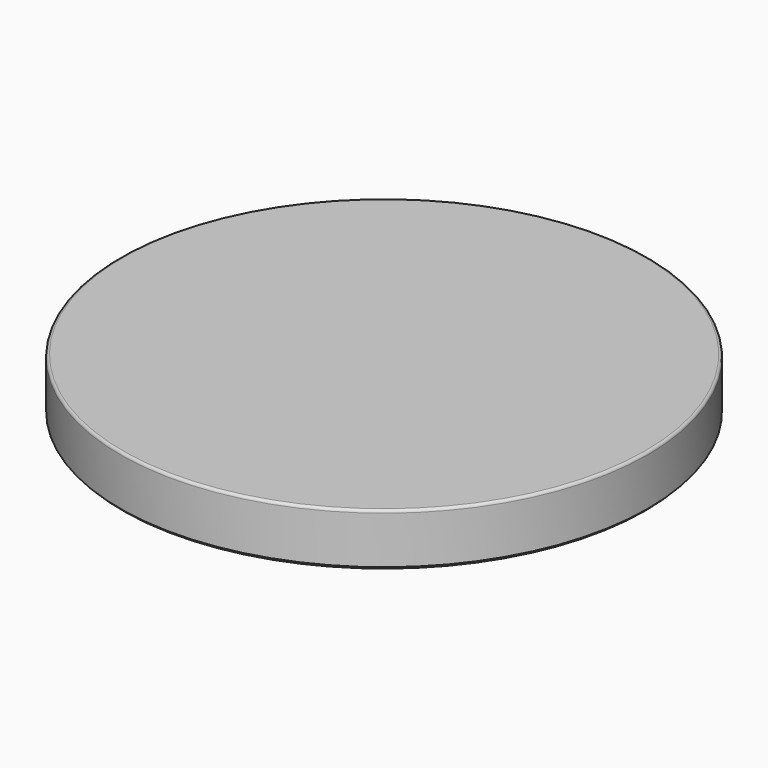
from build123d import *

# Parameters (mm, degrees)
F0_R     = 127
F1_DEPTH = 25.4
F2_R     = 120.65
F2_R_2   = 115.57
F4_DEPTH = 6.35
F3_R     = 22.225
F6_DEPTH = 15.24
F7_D     = 12.7
F7_DEPTH = 12.7
F7_TIP   = 3.8154649308
F8_R     = 1.27
F9_SIZE  = 1.27


with BuildPart() as f1:
    # F0 (on Top) → F1 (new body)
    with BuildSketch(Plane.XY):
        Circle(F0_R)
    extrude(amount=F1_DEPTH)

    # F2 (on face) → F4 (cut)
    with BuildSketch(Plane(origin=(0, 0, 0), x_dir=(1, 0, 0), z_dir=(0, 0, -1))):
        Circle(F2_R)
        Circle(F2_R_2, mode=Mode.SUBTRACT)
    extrude(amount=-F4_DEPTH, mode=Mode.SUBTRACT)

    # F3 (on Top) → F6 (cut)
    with BuildSketch(Plane.XY):
        Circle(F3_R)
    extrude(amount=F6_DEPTH, mode=Mode.SUBTRACT)

    # F7
    with Locations(Plane(origin=(0, 0, 0), x_dir=(1, 0, 0), z_dir=(0, 0, -1))):
        with Locations((31.75, 0), (-31.75, 0)):
            Hole(F7_D / 2, depth=F7_DEPTH)
            with Locations((0, 0, -(F7_DEPTH + F7_TIP / 2))):  # 118° drill point
                Cone(0, F7_D / 2, F7_TIP, mode=Mode.SUBTRACT)

    # F8
    f8_edges = [f1.edges().sort_by_distance(p)[0] for p in [
        (-22.225, 0, 15.24),
        (-127, 0, 25.4),
    ]]
    fillet(f8_edges, radius=F8_R)

    # F9
    f9_edges = [f1.edges().sort_by_distance(p)[0] for p in [
        (-22.225, 0, 0),
        (-115.57, 0, 0),
        (-120.65, 0, 0),
        (-127, 0, 0),
        (-38.1, 0, 0),
        (25.4, 0, 0),
    ]]
    chamfer(f9_edges, length=F9_SIZE)


solid = f1.part
